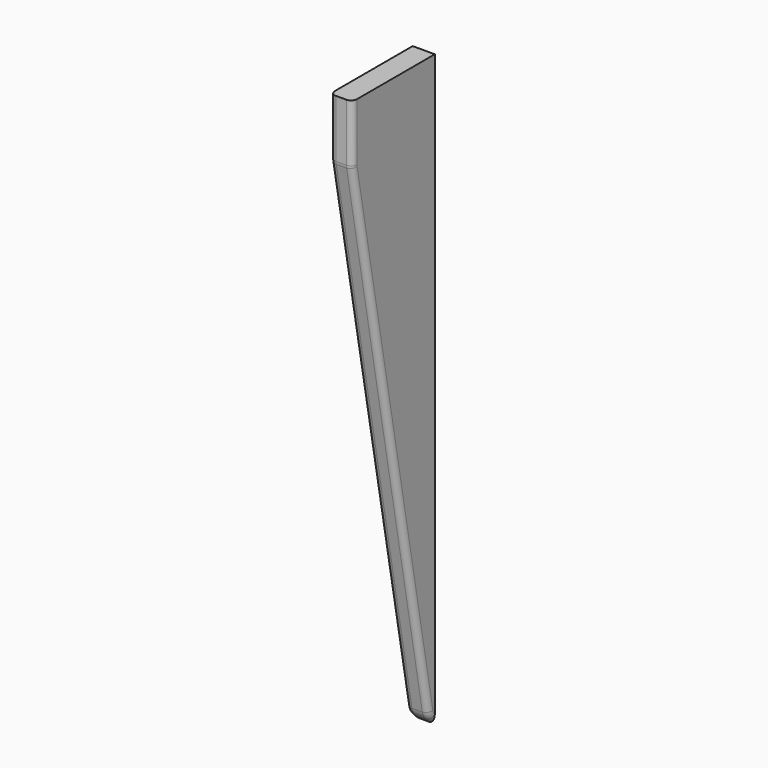
from build123d import *

# Parameters (mm, degrees)
F1_DEPTH     = 19.05
F2_T1_DEPTH  = 453.2334559577
F2_T3_DEPTH  = 17.7217096423
F2_T5_DEPTH  = 62.3469086479
F2_T8_ANGLE  = 10.3758449201
F2_T10_ANGLE = 34.6241550799
F2_T12_ANGLE = 10.3758449201
F2_T14_ANGLE = 34.6241550799


# Not quite as in the source:
# - a fillet or chamfer that OpenCascade refuses, or shapes differently, is made with other operations: its cross-section is extruded or revolved along the edge and cut away or added


with BuildPart() as f1:
    # F0 (on Right) → F1 (new body)
    with BuildSketch(Plane.YZ):
        with BuildLine():
            Line((42.4285726043, -178.7500022879), (42.4285726043, 329.2499977121))
            Line((42.4285726043, 329.2499977121), (-46.4714273957, 329.2499977121))
            Line((-46.4714273957, 329.2499977121), (-46.4714273957, 279.6030890642))
            ThreePointArc((-46.4714273957, 279.6030890642), (-46.4194016068, 278.4547213725), (-46.2637504894, 277.3157623006))
            Line((-46.2637504894, 277.3157623006), (35.3656206904, -168.5061879892))
            ThreePointArc((35.3656206904, -168.5061879892), (36.6122005726, -172.1199848152), (38.877687663, -175.1991173466))
            Line((38.877687663, -175.1991173466), (42.4285726043, -178.7500022879))
        make_face()
    extrude(amount=F1_DEPTH)

    # F2: fillet of radius 5.08 on 2 edges, made by hand

    # F2_s2 → F2_t1 (cut)
    with BuildSketch(Plane(origin=(0, -50.6297547862, 276.5163530631), x_dir=(1, 0, 0), z_dir=(0, 0.1801044696, -0.9836474877))):
        with BuildLine():
            ThreePointArc((13.97, -4.4385863345), (17.5621024484, -5.9264838861), (19.05, -9.5185863345))
            Line((19.05, -9.5185863345), (19.05, -4.4385863345))
            Line((19.05, -4.4385863345), (13.97, -4.4385863345))
        make_face()
        with BuildLine():
            ThreePointArc((5.08, -4.4385863345), (1.4878975516, -5.9264838861), (0, -9.5185863345))
            Line((0, -9.5185863345), (0, -4.4385863345))
            Line((0, -4.4385863345), (5.08, -4.4385863345))
        make_face()
    extrude(amount=F2_T1_DEPTH, mode=Mode.SUBTRACT)

    # F2_s4 → F2_t3 (cut)
    with BuildSketch(Plane(origin=(0, 107.0384025048, -107.0384025048), x_dir=(1, 0, 0), z_dir=(0, 0.7071067812, -0.7071067812))):
        with BuildLine():
            ThreePointArc((5.08, 96.3938073503), (1.4878975516, 94.9059097987), (0, 91.3138073503))
            Line((0, 91.3138073503), (0, 96.3938073503))
            Line((0, 96.3938073503), (5.08, 96.3938073503))
        make_face()
        with BuildLine():
            ThreePointArc((13.97, 96.3938073503), (17.5621024484, 94.9059097987), (19.05, 91.3138073503))
            Line((19.05, 91.3138073503), (19.05, 96.3938073503))
            Line((19.05, 96.3938073503), (13.97, 96.3938073503))
        make_face()
    extrude(amount=F2_T3_DEPTH, mode=Mode.SUBTRACT)

    # F2_s6 → F2_t5 (cut)
    with BuildSketch(Plane.XY.offset(279.6030890642)):
        with BuildLine():
            ThreePointArc((5.08, -46.4714273957), (1.4878975516, -44.9835298442), (0, -41.3914273957))
            Line((0, -41.3914273957), (0, -46.4714273957))
            Line((0, -46.4714273957), (5.08, -46.4714273957))
        make_face()
        with BuildLine():
            ThreePointArc((13.97, -46.4714273957), (17.5621024484, -44.9835298442), (19.05, -41.3914273957))
            Line((19.05, -41.3914273957), (19.05, -46.4714273957))
            Line((19.05, -46.4714273957), (13.97, -46.4714273957))
        make_face()
    extrude(amount=F2_T5_DEPTH, mode=Mode.SUBTRACT)

    # F2_s7 → F2_t8 (revolve, cut)
    with BuildSketch(Plane.XY.offset(279.6030890642)):
        with BuildLine():
            ThreePointArc((5.08, -46.4714273957), (1.4878975516, -44.9835298442), (0, -41.3914273957))
            Line((0, -41.3914273957), (0, -46.4714273957))
            Line((0, -46.4714273957), (5.08, -46.4714273957))
        make_face()
    revolve(axis=Axis((0, -33.7714273957, 279.6030890642), (1, 0, 0)), revolution_arc=F2_T8_ANGLE, mode=Mode.SUBTRACT)

    # F2_s9 → F2_t10 (revolve, cut)
    with BuildSketch(Plane(origin=(0, 30.9996163936, -169.3055972266), x_dir=(1, 0, 0), z_dir=(0, -0.1801044696, 0.9836474877))):
        with BuildLine():
            ThreePointArc((5.08, 4.4385863345), (1.4878975516, 5.9264838861), (0, 9.5185863345))
            Line((0, 9.5185863345), (0, 4.4385863345))
            Line((0, 4.4385863345), (5.08, 4.4385863345))
        make_face()
    revolve(axis=Axis((0, 47.8579437841, -166.2188612255), (1, 0, 0)), revolution_arc=F2_T10_ANGLE, mode=Mode.SUBTRACT)

    # F2_s11 → F2_t12 (revolve, cut)
    with BuildSketch(Plane.XY.offset(279.6030890642)):
        with BuildLine():
            ThreePointArc((13.97, -46.4714273957), (17.5621024484, -44.9835298442), (19.05, -41.3914273957))
            Line((19.05, -41.3914273957), (19.05, -46.4714273957))
            Line((19.05, -46.4714273957), (13.97, -46.4714273957))
        make_face()
    revolve(axis=Axis((19.05, -33.7714273957, 279.6030890642), (1, 0, 0)), revolution_arc=F2_T12_ANGLE, mode=Mode.SUBTRACT)

    # F2_s13 → F2_t14 (revolve, cut)
    with BuildSketch(Plane(origin=(0, 30.9996163936, -169.3055972266), x_dir=(1, 0, 0), z_dir=(0, -0.1801044696, 0.9836474877))):
        with BuildLine():
            ThreePointArc((13.97, 4.4385863345), (17.5621024484, 5.9264838861), (19.05, 9.5185863345))
            Line((19.05, 9.5185863345), (19.05, 4.4385863345))
            Line((19.05, 4.4385863345), (13.97, 4.4385863345))
        make_face()
    revolve(axis=Axis((19.05, 47.8579437841, -166.2188612255), (1, 0, 0)), revolution_arc=F2_T14_ANGLE, mode=Mode.SUBTRACT)


solid = f1.part
